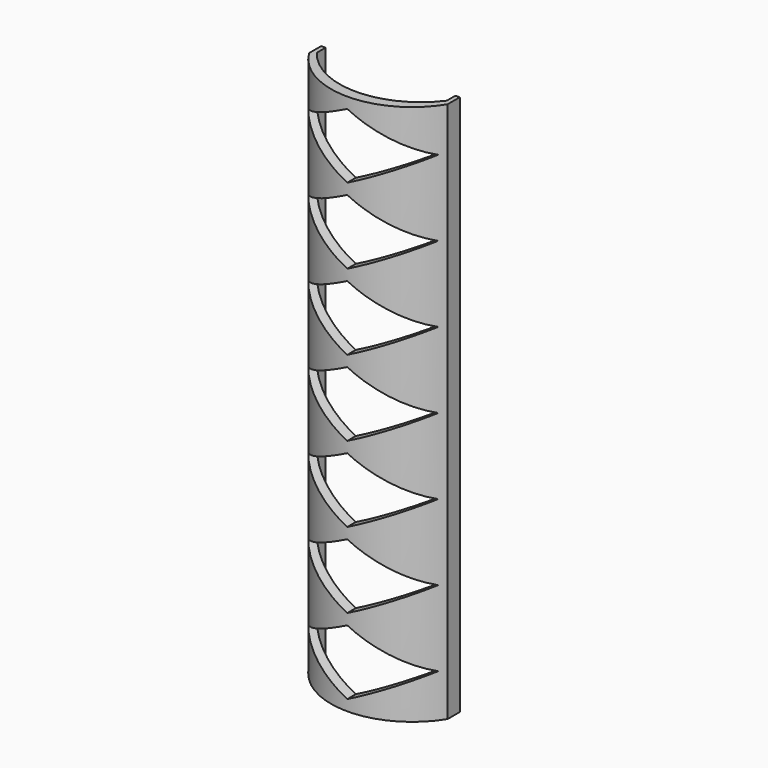
from build123d import *

# Parameters (mm, degrees)
F1_DEPTH = 250
F3_DEPTH = 250
F5_DEPTH = 37.501


# Not quite as in the source:
# - a feature names something its author has since deleted; it is built from what else it names


with BuildPart() as f1:
    # F0 (on Top) → F1 (new body)
    with BuildSketch(Plane.XY):
        with BuildLine():
            Line((-32, -12.551214796), (-32, -19.551214796))
            ThreePointArc((-32, -19.551214796), (0, -37.5), (32, -19.551214796))
            Line((32, -19.551214796), (32, -12.551214796))
            Line((32, -12.551214796), (0, -12.551214796))
            Line((0, -12.551214796), (-32, -12.551214796))
        make_face()
    extrude(amount=F1_DEPTH)

    # F2 (on face) → F3 (cut)
    with BuildSketch(Plane(origin=(0, 0, 0), x_dir=(1, 0, 0), z_dir=(0, 0, -1))):
        with BuildLine():
            Line((-30, 12.551214796), (30, 12.551214796))
            Line((30, 12.551214796), (30, 17.551214796))
            ThreePointArc((30, 17.551214796), (0, 32.551214796), (-30, 17.551214796))
            Line((-30, 17.551214796), (-30, 12.551214796))
        make_face()
    extrude(amount=-F3_DEPTH, mode=Mode.SUBTRACT)

    # F4 (on Front) → F5 (cut, through all)
    with BuildSketch(Plane.XZ):
        Polygon((-30, 20), (0, 5), (30, 20), (0, 35), align=None)
        Polygon((0, 40), (30, 55), (0, 70), (-30, 55), align=None)
        Polygon((0, 110), (30, 125), (0, 140), (-30, 125), align=None)
        Polygon((0, 145), (30, 160), (0, 175), (-30, 160), align=None)
        Polygon((0, 180), (30, 195), (0, 210), (-30, 195), align=None)
        Polygon((0, 215), (30, 230), (0, 245), (-30, 230), align=None)
        Polygon((0, 75), (30, 90), (0, 105), (-30, 90), align=None)
    extrude(amount=F5_DEPTH, mode=Mode.SUBTRACT)


solid = f1.part
